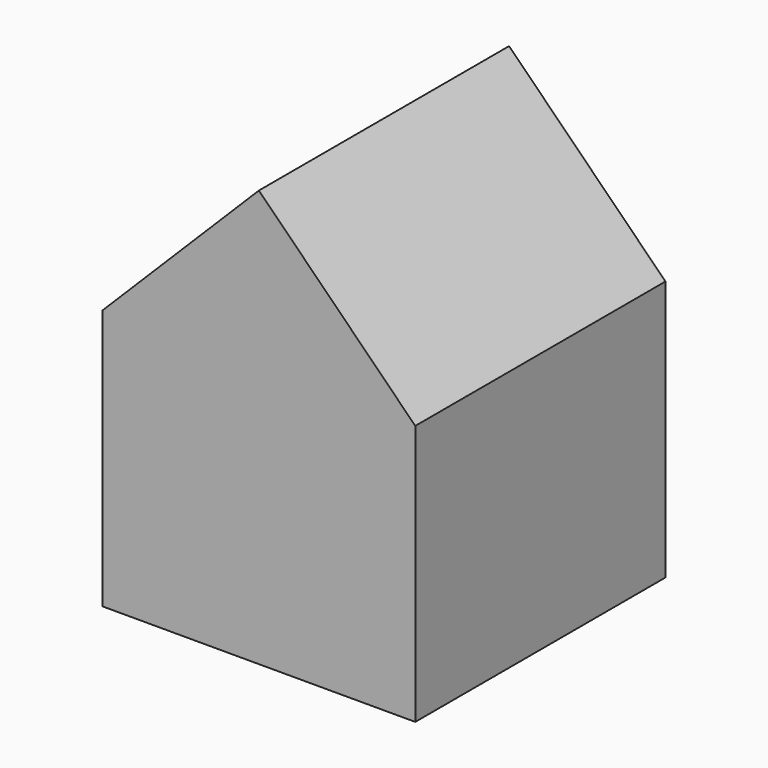
from build123d import *

# Parameters (mm, degrees)
F0_W        = 30
F0_H        = 30
F0_W_2      = 20
F0_H_2      = 20
F1_DEPTH    = 25
F2_W        = 30
F2_H        = 30
F3_DEPTH    = 25
F4_T1_DEPTH = 158.5841493983


# Not quite as in the source:
# - a fillet or chamfer that OpenCascade refuses, or shapes differently, is made with other operations: its cross-section is extruded or revolved along the edge and cut away or added


with BuildPart() as f1:
    # F0 (on Top) → F1 (new body)
    with BuildSketch(Plane.XY):
        with Locations((15, 15)):
            Rectangle(F0_W, F0_H)
        with Locations((15, 15)):
            Rectangle(F0_W_2, F0_H_2, mode=Mode.SUBTRACT)
    extrude(amount=F1_DEPTH)

    # F2 (on face) → F3 (join)
    with BuildSketch(Plane.XY.offset(25)):
        with Locations((15, 15)):
            Rectangle(F2_W, F2_H)
    extrude(amount=F3_DEPTH)

    # F4: chamfer of 25 on 2 edges, made by hand

    # F4_s2 → F4_t1 (cut)
    with BuildSketch(Plane.XZ.offset(-94.2920746991)):
        Polygon((0, 25), (25, 50), (0, 50), align=None)
        Polygon((5, 50), (30, 25), (30, 50), align=None)
    extrude(amount=F4_T1_DEPTH, mode=Mode.SUBTRACT)


solid = f1.part
